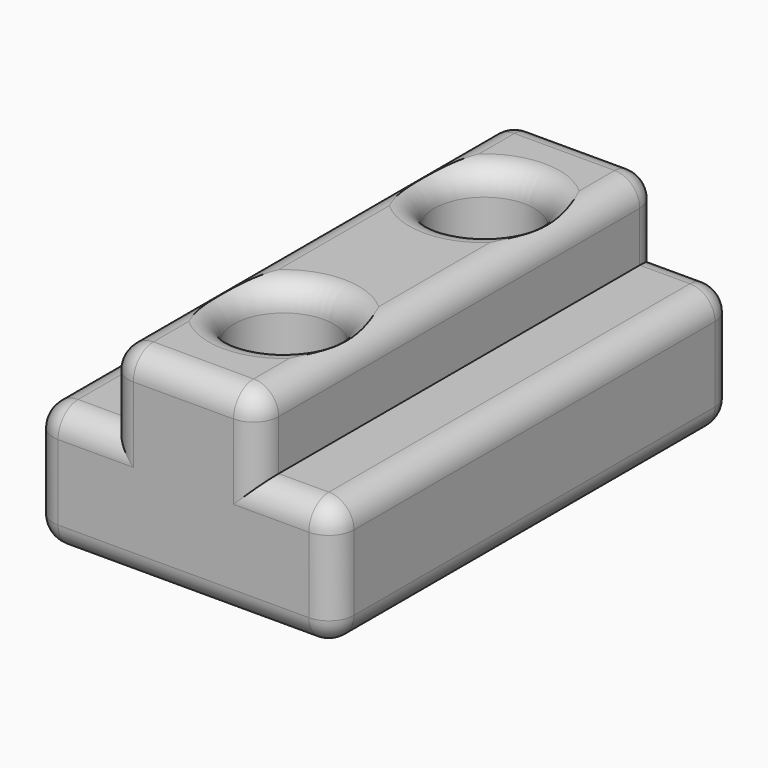
from build123d import *

# Parameters (mm, degrees)
F1_DEPTH      = 20
F2_R          = 2
F3_DEPTH      = 8.001
F4_T1_DEPTH   = 18
F4_T3_DEPTH   = 4
F4_T5_DEPTH   = 3
F4_T7_DEPTH   = 10
F4_T9_DEPTH   = 2
F4_T11_DEPTH  = 2
F4_T13_DEPTH  = 2
F4_S17_W      = 1
F4_S17_H      = 1
F4_T18_DEPTH  = 1
F4_S23_W      = 1
F4_S23_H      = 1
F4_T24_DEPTH  = 1
F4_S29_W      = 1
F4_S29_H      = 1
F4_T30_DEPTH  = 1
F4_S35_W      = 1
F4_S35_H      = 1
F4_T36_DEPTH  = 1
F4_S41_W      = 1
F4_S41_H      = 1
F4_T42_DEPTH  = 1
F4_S47_W      = 1
F4_S47_H      = 1
F4_T48_DEPTH  = 1
F4_S53_W      = 1
F4_S53_H      = 1
F4_T54_DEPTH  = 1
F4_S59_W      = 1
F4_S59_H      = 1
F4_T60_DEPTH  = 1
F4_S65_W      = 1
F4_S65_H      = 1
F4_T66_DEPTH  = 1
F4_S71_W      = 1
F4_S71_H      = 1
F4_T72_DEPTH  = 1
F4_S77_W      = 1
F4_S77_H      = 1
F4_T78_DEPTH  = 1
F4_S83_W      = 1
F4_S83_H      = 1
F4_T84_DEPTH  = 1
F4_T95_DEPTH  = 4.5
F4_T99_DEPTH  = 4.5
F4_T106_DEPTH = 4.5
F4_T110_DEPTH = 4.5
F4_T117_DEPTH = 4.5
F4_T121_DEPTH = 4.5
F4_T128_DEPTH = 4.5
F4_T132_DEPTH = 4.5


# Not quite as in the source:
# - a fillet or chamfer that OpenCascade refuses, or shapes differently, is made with other operations: its cross-section is extruded or revolved along the edge and cut away or added


with BuildPart() as f1:
    # F0 (on Front) → F1 (new body)
    with BuildSketch(Plane.XZ):
        Polygon((0, 5), (0, 0), (12, 0), (12, 5), (9, 5), (9, 8), (3, 8), (3, 5), align=None)
    extrude(amount=F1_DEPTH)

    # F2 (on face) → F3 (cut, through all)
    with BuildSketch(Plane.XY.offset(8)):
        with Locations((6, -5)):
            Circle(F2_R)
        with Locations((6, -15)):
            Circle(F2_R)
    extrude(amount=-F3_DEPTH, mode=Mode.SUBTRACT)

    # F4: fillet of radius 1 on 24 edges, made by hand

    # F4_s2 → F4_t1 (cut)
    with BuildSketch(Plane.XZ.offset(1)):
        with BuildLine():
            ThreePointArc((9, 7), (8.7071067812, 7.7071067812), (8, 8))
            Line((8, 8), (9, 8))
            Line((9, 8), (9, 7))
        make_face()
        with BuildLine():
            ThreePointArc((3, 7), (3.2928932188, 7.7071067812), (4, 8))
            Line((4, 8), (3, 8))
            Line((3, 8), (3, 7))
        make_face()
        with BuildLine():
            ThreePointArc((11, 0), (11.7071067812, 0.2928932188), (12, 1))
            Line((12, 1), (12, 0))
            Line((12, 0), (11, 0))
        make_face()
        with BuildLine():
            ThreePointArc((12, 4), (11.7071067812, 4.7071067812), (11, 5))
            Line((11, 5), (12, 5))
            Line((12, 5), (12, 4))
        make_face()
        with BuildLine():
            ThreePointArc((0, 4), (0.2928932188, 4.7071067812), (1, 5))
            Line((1, 5), (0, 5))
            Line((0, 5), (0, 4))
        make_face()
        with BuildLine():
            ThreePointArc((0, 1), (0.2928932188, 0.2928932188), (1, 0))
            Line((1, 0), (0, 0))
            Line((0, 0), (0, 1))
        make_face()
    extrude(amount=F4_T1_DEPTH, mode=Mode.SUBTRACT)

    # F4_s4 → F4_t3 (cut)
    with BuildSketch(Plane.YZ.offset(4)):
        with BuildLine():
            ThreePointArc((0, 7), (-0.2928932188, 7.7071067812), (-1, 8))
            Line((-1, 8), (0, 8))
            Line((0, 8), (0, 7))
        make_face()
        with BuildLine():
            ThreePointArc((-20, 7), (-19.7071067812, 7.7071067812), (-19, 8))
            Line((-19, 8), (-20, 8))
            Line((-20, 8), (-20, 7))
        make_face()
    extrude(amount=F4_T3_DEPTH, mode=Mode.SUBTRACT)

    # F4_s6 → F4_t5 (cut)
    with BuildSketch(Plane.XY.offset(1)):
        with BuildLine():
            ThreePointArc((11, 0), (11.7071067812, -0.2928932188), (12, -1))
            Line((12, -1), (12, 0))
            Line((12, 0), (11, 0))
        make_face()
        with BuildLine():
            ThreePointArc((11, -20), (11.7071067812, -19.7071067812), (12, -19))
            Line((12, -19), (12, -20))
            Line((12, -20), (11, -20))
        make_face()
        with BuildLine():
            ThreePointArc((0, -1), (0.2928932188, -0.2928932188), (1, 0))
            Line((1, 0), (0, 0))
            Line((0, 0), (0, -1))
        make_face()
        with BuildLine():
            ThreePointArc((0, -19), (0.2928932188, -19.7071067812), (1, -20))
            Line((1, -20), (0, -20))
            Line((0, -20), (0, -19))
        make_face()
    extrude(amount=F4_T5_DEPTH, mode=Mode.SUBTRACT)

    # F4_s8 → F4_t7 (cut)
    with BuildSketch(Plane.YZ.offset(1)):
        with BuildLine():
            ThreePointArc((-19, 0), (-19.7071067812, 0.2928932188), (-20, 1))
            Line((-20, 1), (-20, 0))
            Line((-20, 0), (-19, 0))
        make_face()
        with BuildLine():
            ThreePointArc((-1, 0), (-0.2928932188, 0.2928932188), (0, 1))
            Line((0, 1), (0, 0))
            Line((0, 0), (-1, 0))
        make_face()
    extrude(amount=F4_T7_DEPTH, mode=Mode.SUBTRACT)

    # F4_s10 → F4_t9 (cut)
    with BuildSketch(Plane.YZ.offset(9)):
        with BuildLine():
            ThreePointArc((-20, 4), (-19.7071067812, 4.7071067812), (-19, 5))
            Line((-19, 5), (-20, 5))
            Line((-20, 5), (-20, 4))
        make_face()
        with BuildLine():
            ThreePointArc((0, 4), (-0.2928932188, 4.7071067812), (-1, 5))
            Line((-1, 5), (0, 5))
            Line((0, 5), (0, 4))
        make_face()
    extrude(amount=F4_T9_DEPTH, mode=Mode.SUBTRACT)

    # F4_s12 → F4_t11 (cut)
    with BuildSketch(Plane.XY.offset(5)):
        with BuildLine():
            ThreePointArc((8, -20), (8.7071067812, -19.7071067812), (9, -19))
            Line((9, -19), (9, -20))
            Line((9, -20), (8, -20))
        make_face()
        with BuildLine():
            ThreePointArc((4, -20), (3.2928932188, -19.7071067812), (3, -19))
            Line((3, -19), (3, -20))
            Line((3, -20), (4, -20))
        make_face()
        with BuildLine():
            ThreePointArc((8, 0), (8.7071067812, -0.2928932188), (9, -1))
            Line((9, -1), (9, 0))
            Line((9, 0), (8, 0))
        make_face()
        with BuildLine():
            ThreePointArc((4, 0), (3.2928932188, -0.2928932188), (3, -1))
            Line((3, -1), (3, 0))
            Line((3, 0), (4, 0))
        make_face()
    extrude(amount=F4_T11_DEPTH, mode=Mode.SUBTRACT)

    # F4_s14 → F4_t13 (cut)
    with BuildSketch(Plane.YZ.offset(1)):
        with BuildLine():
            ThreePointArc((-19, 5), (-19.7071067812, 4.7071067812), (-20, 4))
            Line((-20, 4), (-20, 5))
            Line((-20, 5), (-19, 5))
        make_face()
        with BuildLine():
            ThreePointArc((-1, 5), (-0.2928932188, 4.7071067812), (0, 4))
            Line((0, 4), (0, 5))
            Line((0, 5), (-1, 5))
        make_face()
    extrude(amount=F4_T13_DEPTH, mode=Mode.SUBTRACT)


with BuildPart() as f4_tool16:
    # F4_s17 → F4_t18 (new body)
    with BuildSketch(Plane.XZ.offset(1)):
        with Locations((8.5, 7.5)):
            Rectangle(F4_S17_W, F4_S17_H)
    extrude(amount=-F4_T18_DEPTH)

    # F4_s19 → F4_t20 (revolve, cut)
    with BuildSketch(Plane(origin=(8, -1, 7), x_dir=(-0.7071067812, 0, -0.7071067812), z_dir=(0.7071067812, 0, -0.7071067812))):
        with BuildLine():
            ThreePointArc((0, -1), (1, 0), (0, 1))
            Line((0, 1), (0, -1))
        make_face()
    revolve(axis=Axis((8, -1, 7), (0, 1, 0)), mode=Mode.SUBTRACT)


with BuildPart() as f1_1:
    add(f1.part)

    # F4_t15: cut F4_tool16
    add(f4_tool16.part, mode=Mode.SUBTRACT)


with BuildPart() as f4_tool22:
    # F4_s23 → F4_t24 (new body)
    with BuildSketch(Plane.YZ.offset(8)):
        with Locations((-19.5, 7.5)):
            Rectangle(F4_S23_W, F4_S23_H)
    extrude(amount=F4_T24_DEPTH)

    # F4_s25 → F4_t26 (revolve, cut)
    with BuildSketch(Plane(origin=(8, -19, 7), x_dir=(0, 0.7071067812, -0.7071067812), z_dir=(0, -0.7071067812, -0.7071067812))):
        with BuildLine():
            ThreePointArc((0, -1), (1, 0), (0, 1))
            Line((0, 1), (0, -1))
        make_face()
    revolve(axis=Axis((8, -19, 7), (1, 0, 0)), mode=Mode.SUBTRACT)


with BuildPart() as f1_2:
    add(f1_1.part)

    # F4_t21: cut F4_tool22
    add(f4_tool22.part, mode=Mode.SUBTRACT)


with BuildPart() as f4_tool28:
    # F4_s29 → F4_t30 (new body)
    with BuildSketch(Plane.XY.offset(7)):
        with Locations((3.5, -0.5)):
            Rectangle(F4_S29_W, F4_S29_H)
    extrude(amount=F4_T30_DEPTH)

    # F4_s31 → F4_t32 (revolve, cut)
    with BuildSketch(Plane(origin=(4, -1, 7), x_dir=(0.7071067812, -0.7071067812, 0), z_dir=(-0.7071067812, -0.7071067812, 0))):
        with BuildLine():
            ThreePointArc((0, -1), (1, 0), (0, 1))
            Line((0, 1), (0, -1))
        make_face()
    revolve(axis=Axis((4, -1, 7), (0, 0, 1)), mode=Mode.SUBTRACT)


with BuildPart() as f1_3:
    add(f1_2.part)

    # F4_t27: cut F4_tool28
    add(f4_tool28.part, mode=Mode.SUBTRACT)


with BuildPart() as f4_tool34:
    # F4_s35 → F4_t36 (new body)
    with BuildSketch(Plane.XY.offset(7)):
        with Locations((3.5, -19.5)):
            Rectangle(F4_S35_W, F4_S35_H)
    extrude(amount=F4_T36_DEPTH)

    # F4_s37 → F4_t38 (revolve, cut)
    with BuildSketch(Plane(origin=(4, -19, 7), x_dir=(0.7071067812, 0.7071067812, 0), z_dir=(0.7071067812, -0.7071067812, 0))):
        with BuildLine():
            ThreePointArc((0, -1), (1, 0), (0, 1))
            Line((0, 1), (0, -1))
        make_face()
    revolve(axis=Axis((4, -19, 7), (0, 0, 1)), mode=Mode.SUBTRACT)


with BuildPart() as f1_4:
    add(f1_3.part)

    # F4_t33: cut F4_tool34
    add(f4_tool34.part, mode=Mode.SUBTRACT)


with BuildPart() as f4_tool40:
    # F4_s41 → F4_t42 (new body)
    with BuildSketch(Plane.XY.offset(1)):
        with Locations((11.5, -0.5)):
            Rectangle(F4_S41_W, F4_S41_H)
    extrude(amount=-F4_T42_DEPTH)

    # F4_s43 → F4_t44 (revolve, cut)
    with BuildSketch(Plane(origin=(11, -1, 1), x_dir=(-0.7071067812, -0.7071067812, 0), z_dir=(0.7071067812, -0.7071067812, 0))):
        with BuildLine():
            ThreePointArc((0, -1), (1, 0), (0, 1))
            Line((0, 1), (0, -1))
        make_face()
    revolve(axis=Axis((11, -1, 1), (0, 0, -1)), mode=Mode.SUBTRACT)


with BuildPart() as f1_5:
    add(f1_4.part)

    # F4_t39: cut F4_tool40
    add(f4_tool40.part, mode=Mode.SUBTRACT)


with BuildPart() as f4_tool46:
    # F4_s47 → F4_t48 (new body)
    with BuildSketch(Plane.XY.offset(1)):
        with Locations((11.5, -19.5)):
            Rectangle(F4_S47_W, F4_S47_H)
    extrude(amount=-F4_T48_DEPTH)

    # F4_s49 → F4_t50 (revolve, cut)
    with BuildSketch(Plane(origin=(11, -19, 1), x_dir=(-0.7071067812, 0.7071067812, 0), z_dir=(-0.7071067812, -0.7071067812, 0))):
        with BuildLine():
            ThreePointArc((0, -1), (1, 0), (0, 1))
            Line((0, 1), (0, -1))
        make_face()
    revolve(axis=Axis((11, -19, 1), (0, 0, -1)), mode=Mode.SUBTRACT)


with BuildPart() as f1_6:
    add(f1_5.part)

    # F4_t45: cut F4_tool46
    add(f4_tool46.part, mode=Mode.SUBTRACT)


with BuildPart() as f4_tool52:
    # F4_s53 → F4_t54 (new body)
    with BuildSketch(Plane.XY.offset(4)):
        with Locations((11.5, -0.5)):
            Rectangle(F4_S53_W, F4_S53_H)
    extrude(amount=F4_T54_DEPTH)

    # F4_s55 → F4_t56 (revolve, cut)
    with BuildSketch(Plane(origin=(11, -1, 4), x_dir=(-0.7071067812, -0.7071067812, 0), z_dir=(-0.7071067812, 0.7071067812, 0))):
        with BuildLine():
            ThreePointArc((0, -1), (1, 0), (0, 1))
            Line((0, 1), (0, -1))
        make_face()
    revolve(axis=Axis((11, -1, 4), (0, 0, 1)), mode=Mode.SUBTRACT)


with BuildPart() as f1_7:
    add(f1_6.part)

    # F4_t51: cut F4_tool52
    add(f4_tool52.part, mode=Mode.SUBTRACT)


with BuildPart() as f4_tool58:
    # F4_s59 → F4_t60 (new body)
    with BuildSketch(Plane.XY.offset(4)):
        with Locations((11.5, -19.5)):
            Rectangle(F4_S59_W, F4_S59_H)
    extrude(amount=F4_T60_DEPTH)

    # F4_s61 → F4_t62 (revolve, cut)
    with BuildSketch(Plane(origin=(11, -19, 4), x_dir=(-0.7071067812, 0.7071067812, 0), z_dir=(0.7071067812, 0.7071067812, 0))):
        with BuildLine():
            ThreePointArc((0, -1), (1, 0), (0, 1))
            Line((0, 1), (0, -1))
        make_face()
    revolve(axis=Axis((11, -19, 4), (0, 0, 1)), mode=Mode.SUBTRACT)


with BuildPart() as f1_8:
    add(f1_7.part)

    # F4_t57: cut F4_tool58
    add(f4_tool58.part, mode=Mode.SUBTRACT)


with BuildPart() as f4_tool64:
    # F4_s65 → F4_t66 (new body)
    with BuildSketch(Plane.YZ.offset(1)):
        with Locations((-0.5, 4.5)):
            Rectangle(F4_S65_W, F4_S65_H)
    extrude(amount=-F4_T66_DEPTH)

    # F4_s67 → F4_t68 (revolve, cut)
    with BuildSketch(Plane(origin=(1, -1, 4), x_dir=(0, -0.7071067812, -0.7071067812), z_dir=(0, 0.7071067812, -0.7071067812))):
        with BuildLine():
            ThreePointArc((0, -1), (1, 0), (0, 1))
            Line((0, 1), (0, -1))
        make_face()
    revolve(axis=Axis((1, -1, 4), (-1, 0, 0)), mode=Mode.SUBTRACT)


with BuildPart() as f1_9:
    add(f1_8.part)

    # F4_t63: cut F4_tool64
    add(f4_tool64.part, mode=Mode.SUBTRACT)


with BuildPart() as f4_tool70:
    # F4_s71 → F4_t72 (new body)
    with BuildSketch(Plane.YZ.offset(1)):
        with Locations((-19.5, 4.5)):
            Rectangle(F4_S71_W, F4_S71_H)
    extrude(amount=-F4_T72_DEPTH)

    # F4_s73 → F4_t74 (revolve, cut)
    with BuildSketch(Plane(origin=(1, -19, 4), x_dir=(0, 0.7071067812, -0.7071067812), z_dir=(0, 0.7071067812, 0.7071067812))):
        with BuildLine():
            ThreePointArc((0, -1), (1, 0), (0, 1))
            Line((0, 1), (0, -1))
        make_face()
    revolve(axis=Axis((1, -19, 4), (-1, 0, 0)), mode=Mode.SUBTRACT)


with BuildPart() as f1_10:
    add(f1_9.part)

    # F4_t69: cut F4_tool70
    add(f4_tool70.part, mode=Mode.SUBTRACT)


with BuildPart() as f4_tool76:
    # F4_s77 → F4_t78 (new body)
    with BuildSketch(Plane.YZ.offset(1)):
        with Locations((-0.5, 0.5)):
            Rectangle(F4_S77_W, F4_S77_H)
    extrude(amount=-F4_T78_DEPTH)

    # F4_s79 → F4_t80 (revolve, cut)
    with BuildSketch(Plane(origin=(1, -1, 1), x_dir=(0, -0.7071067812, 0.7071067812), z_dir=(0, -0.7071067812, -0.7071067812))):
        with BuildLine():
            ThreePointArc((0, -1), (1, 0), (0, 1))
            Line((0, 1), (0, -1))
        make_face()
    revolve(axis=Axis((1, -1, 1), (-1, 0, 0)), mode=Mode.SUBTRACT)


with BuildPart() as f1_11:
    add(f1_10.part)

    # F4_t75: cut F4_tool76
    add(f4_tool76.part, mode=Mode.SUBTRACT)


with BuildPart() as f4_tool82:
    # F4_s83 → F4_t84 (new body)
    with BuildSketch(Plane.YZ.offset(1)):
        with Locations((-19.5, 0.5)):
            Rectangle(F4_S83_W, F4_S83_H)
    extrude(amount=-F4_T84_DEPTH)

    # F4_s85 → F4_t86 (revolve, cut)
    with BuildSketch(Plane(origin=(1, -19, 1), x_dir=(0, 0.7071067812, 0.7071067812), z_dir=(0, -0.7071067812, 0.7071067812))):
        with BuildLine():
            ThreePointArc((0, -1), (1, 0), (0, 1))
            Line((0, 1), (0, -1))
        make_face()
    revolve(axis=Axis((1, -19, 1), (-1, 0, 0)), mode=Mode.SUBTRACT)


with BuildPart() as f1_12:
    add(f1_11.part)

    # F4_t81: cut F4_tool82
    add(f4_tool82.part, mode=Mode.SUBTRACT)

    # F4_s87 → F4_t88 (revolve, cut)
    with BuildSketch(Plane.XZ.offset(15)):
        with BuildLine():
            ThreePointArc((8, 7), (8.2928932188, 7.7071067812), (9, 8))
            Line((9, 8), (8, 8))
            Line((8, 8), (8, 7))
        make_face()
    revolve(axis=Axis((6, -15, 8), (0, 0, 1)), mode=Mode.SUBTRACT)

    # F4_s89 → F4_t90 (revolve, cut)
    with BuildSketch(Plane.XZ.offset(5)):
        with BuildLine():
            ThreePointArc((8, 7), (8.2928932188, 7.7071067812), (9, 8))
            Line((9, 8), (8, 8))
            Line((8, 8), (8, 7))
        make_face()
    revolve(axis=Axis((6, -5, 8), (0, 0, 1)), mode=Mode.SUBTRACT)


with BuildPart() as f4_tool93:
    # F4_s94 → F4_t95 (new body)
    with BuildSketch(Plane.YZ.offset(11)):
        with BuildLine():
            ThreePointArc((-20, 4), (-19.7071067812, 4.7071067812), (-19, 5))
            Line((-19, 5), (-20, 5))
            Line((-20, 5), (-20, 4))
        make_face()
    extrude(amount=-F4_T95_DEPTH)

    split(bisect_by=Plane.YZ.offset(9), keep=Keep.BOTTOM)


with BuildPart() as f4_tool97:
    # F4_s98 → F4_t99 (new body)
    with BuildSketch(Plane.XY.offset(2.5)):
        with BuildLine():
            ThreePointArc((8, -20), (8.7071067812, -19.7071067812), (9, -19))
            Line((9, -19), (9, -20))
            Line((9, -20), (8, -20))
        make_face()
    extrude(amount=F4_T99_DEPTH)

    split(bisect_by=Plane.XY.offset(5), keep=Keep.BOTTOM)


with BuildPart() as f4_tool93_1:
    add(f4_tool93.part)

    # F4_t101: intersect F4_tool97
    add(f4_tool97.part, mode=Mode.INTERSECT)


with BuildPart() as f1_13:
    add(f1_12.part)

    # F4_t91: cut F4_tool93
    add(f4_tool93_1.part, mode=Mode.SUBTRACT)


with BuildPart() as f4_tool104:
    # F4_s105 → F4_t106 (new body)
    with BuildSketch(Plane.YZ.offset(5.5)):
        with BuildLine():
            ThreePointArc((-19, 5), (-19.7071067812, 4.7071067812), (-20, 4))
            Line((-20, 4), (-20, 5))
            Line((-20, 5), (-19, 5))
        make_face()
    extrude(amount=-F4_T106_DEPTH)

    split(bisect_by=Plane.YZ.offset(3), keep=Keep.TOP)


with BuildPart() as f4_tool108:
    # F4_s109 → F4_t110 (new body)
    with BuildSketch(Plane.XY.offset(7)):
        with BuildLine():
            ThreePointArc((4, -20), (3.2928932188, -19.7071067812), (3, -19))
            Line((3, -19), (3, -20))
            Line((3, -20), (4, -20))
        make_face()
    extrude(amount=-F4_T110_DEPTH)

    split(bisect_by=Plane.XY.offset(5), keep=Keep.BOTTOM)


with BuildPart() as f4_tool104_1:
    add(f4_tool104.part)

    # F4_t112: intersect F4_tool108
    add(f4_tool108.part, mode=Mode.INTERSECT)


with BuildPart() as f1_14:
    add(f1_13.part)

    # F4_t102: cut F4_tool104
    add(f4_tool104_1.part, mode=Mode.SUBTRACT)


with BuildPart() as f4_tool115:
    # F4_s116 → F4_t117 (new body)
    with BuildSketch(Plane.YZ.offset(11)):
        with BuildLine():
            ThreePointArc((0, 4), (-0.2928932188, 4.7071067812), (-1, 5))
            Line((-1, 5), (0, 5))
            Line((0, 5), (0, 4))
        make_face()
    extrude(amount=-F4_T117_DEPTH)

    split(bisect_by=Plane.YZ.offset(9), keep=Keep.BOTTOM)


with BuildPart() as f4_tool119:
    # F4_s120 → F4_t121 (new body)
    with BuildSketch(Plane.XY.offset(2.5)):
        with BuildLine():
            ThreePointArc((8, 0), (8.7071067812, -0.2928932188), (9, -1))
            Line((9, -1), (9, 0))
            Line((9, 0), (8, 0))
        make_face()
    extrude(amount=F4_T121_DEPTH)

    split(bisect_by=Plane.XY.offset(5), keep=Keep.BOTTOM)


with BuildPart() as f4_tool115_1:
    add(f4_tool115.part)

    # F4_t123: intersect F4_tool119
    add(f4_tool119.part, mode=Mode.INTERSECT)


with BuildPart() as f1_15:
    add(f1_14.part)

    # F4_t113: cut F4_tool115
    add(f4_tool115_1.part, mode=Mode.SUBTRACT)


with BuildPart() as f4_tool126:
    # F4_s127 → F4_t128 (new body)
    with BuildSketch(Plane.YZ.offset(5.5)):
        with BuildLine():
            ThreePointArc((-1, 5), (-0.2928932188, 4.7071067812), (0, 4))
            Line((0, 4), (0, 5))
            Line((0, 5), (-1, 5))
        make_face()
    extrude(amount=-F4_T128_DEPTH)

    split(bisect_by=Plane.YZ.offset(3), keep=Keep.TOP)


with BuildPart() as f4_tool130:
    # F4_s131 → F4_t132 (new body)
    with BuildSketch(Plane.XY.offset(7)):
        with BuildLine():
            ThreePointArc((4, 0), (3.2928932188, -0.2928932188), (3, -1))
            Line((3, -1), (3, 0))
            Line((3, 0), (4, 0))
        make_face()
    extrude(amount=-F4_T132_DEPTH)

    split(bisect_by=Plane.XY.offset(5), keep=Keep.BOTTOM)


with BuildPart() as f4_tool126_1:
    add(f4_tool126.part)

    # F4_t134: intersect F4_tool130
    add(f4_tool130.part, mode=Mode.INTERSECT)


with BuildPart() as f1_16:
    add(f1_15.part)

    # F4_t124: cut F4_tool126
    add(f4_tool126_1.part, mode=Mode.SUBTRACT)


solid = f1_16.part
